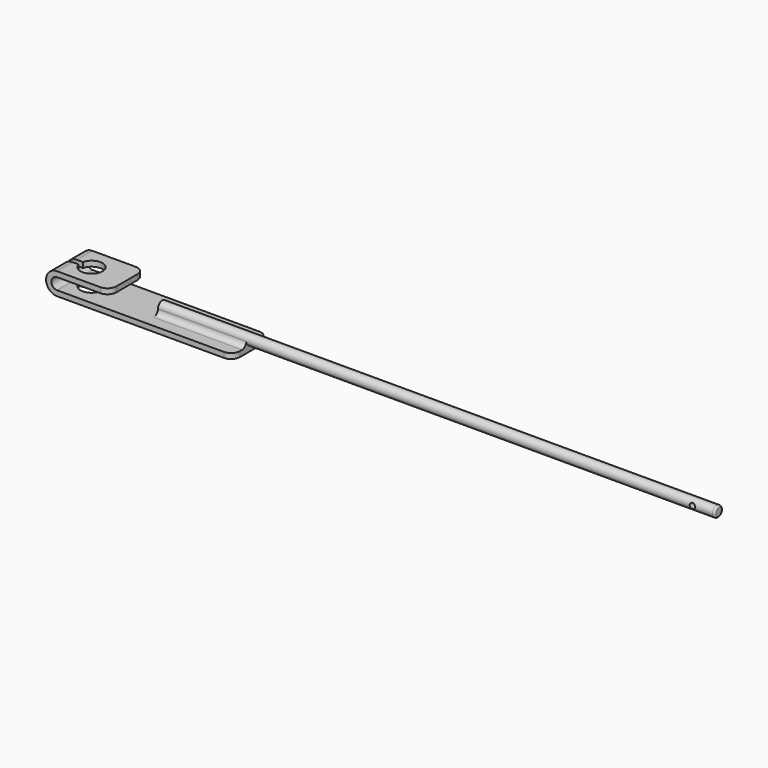
from build123d import *

# Parameters (mm, degrees)
F1_DEPTH      = 25
F3_DEPTH      = 12.501
F4_DEPTH      = 12.501
F7_DEPTH      = 270
F7_DEPTH_BACK = 45
F8_T1_DEPTH   = 45
F8_T3_DEPTH   = 5
F9_R          = 5
F10_R         = 1
F12_D         = 3


# Not quite as in the source:
# - a fillet or chamfer that OpenCascade refuses, or shapes differently, is made with other operations: its cross-section is extruded or revolved along the edge and cut away or added


with BuildPart() as f1:
    # F0 (on Front) → F1 (new body)
    with BuildSketch(Plane.XZ):
        with BuildLine():
            ThreePointArc((-35.5866095653, 3), (-41.8366095653, -3.25), (-35.5866095653, -9.5))
            Line((-35.5866095653, -9.5), (63.9133904347, -9.5))
            Line((63.9133904347, -9.5), (63.9133904347, -6.5))
            Line((63.9133904347, -6.5), (-35.5866095653, -6.5))
            ThreePointArc((-35.5866095653, -6.5), (-38.8366095653, -3.25), (-35.5866095653, 0))
            Line((-35.5866095653, 0), (-6.0866095653, 0))
            Line((-6.0866095653, 0), (-6.0866095653, 3))
            Line((-6.0866095653, 3), (-35.5866095653, 3))
        make_face()
    extrude(amount=F1_DEPTH)

    # F2 (on face) → F3 (cut, through all)
    with BuildSketch(Plane.XY.offset(3)):
        with BuildLine():
            ThreePointArc((-32.153940115, -14), (-25.3310686782, -18.7041645665), (-19.8366095653, -12.5))
            ThreePointArc((-19.8366095653, -12.5), (-25.3310686782, -6.2958354335), (-32.153940115, -11))
            ThreePointArc((-32.153940115, -11), (-32.3366095653, -12.5), (-32.153940115, -14))
        make_face()
    extrude(amount=-F3_DEPTH, mode=Mode.SUBTRACT)

    # F2 (on face) → F4 (cut, through all)
    with BuildSketch(Plane.XY.offset(3)):
        with BuildLine():
            ThreePointArc((-32.153940115, -14), (-25.3310686782, -18.7041645665), (-19.8366095653, -12.5))
            ThreePointArc((-19.8366095653, -12.5), (-25.3310686782, -6.2958354335), (-32.153940115, -11))
            ThreePointArc((-32.153940115, -11), (-32.3366095653, -12.5), (-32.153940115, -14))
        make_face()
        with BuildLine():
            ThreePointArc((-32.153940115, -14), (-32.3366095653, -12.5), (-32.153940115, -11))
            Line((-32.153940115, -11), (-41.9135839269, -11))
            Line((-41.9135839269, -11), (-41.9135839269, -14))
            Line((-41.9135839269, -14), (-32.153940115, -14))
        make_face()
    extrude(amount=-F4_DEPTH, mode=Mode.SUBTRACT)

    # F6 (on offset) → F7 (join, two sides)
    with BuildSketch(Plane.YZ.offset(58.9133904347)) as f7_sk:
        with BuildLine():
            ThreePointArc((-12.4225467883, -6.5), (-10.3514703126, -5.5947574316), (-9.5, -3.501))
            ThreePointArc((-9.5, -3.501), (-14.5937574316, -1.3524703126), (-12.5774532117, -6.5))
            Line((-12.5774532117, -6.5), (-12.4225467883, -6.5))
        make_face()
        with BuildLine():
            Line((-12.4225467883, -6.5), (-12.5774532117, -6.5))
            ThreePointArc((-12.5774532117, -6.5), (-12.5, -6.501), (-12.4225467883, -6.5))
        make_face()
    extrude(amount=F7_DEPTH)
    extrude(f7_sk.sketch, amount=-F7_DEPTH_BACK)

    # F8: fillet of radius 3 on 4 edges, made by hand

    # F8_s2 → F8_t1 (join)
    with BuildSketch(Plane.YZ.offset(13.9133904347)):
        with BuildLine():
            ThreePointArc((-18.5001459648, -6.5004), (-16.3786421293, -5.6217630236), (-15.4995999453, -3.5004270532))
            Line((-15.4995999453, -3.5004270532), (-15.1995453433, -3.500484366))
            ThreePointArc((-15.1995453433, -3.500484366), (-14.4336951193, -5.3852845615), (-12.5697064807, -6.2000454108))
            Line((-12.5697064807, -6.2000454108), (-12.5774532117, -6.8000546074))
            ThreePointArc((-12.5774532117, -6.8000546074), (-15.5387995882, -6.8000546074), (-18.5001459648, -6.8004546074))
            Line((-18.5001459648, -6.8004546074), (-18.5001459648, -6.5004))
        make_face()
        with BuildLine():
            ThreePointArc((-6.4998540352, -6.5004), (-8.6213578707, -5.6217630236), (-9.5004000547, -3.5004270532))
            Line((-9.5004000547, -3.5004270532), (-9.8004546567, -3.500484366))
            ThreePointArc((-9.8004546567, -3.500484366), (-10.5663048807, -5.3852845615), (-12.4302935193, -6.2000454108))
            Line((-12.4302935193, -6.2000454108), (-12.4225467883, -6.8000546074))
            ThreePointArc((-12.4225467883, -6.8000546074), (-9.4612004118, -6.8000546074), (-6.4998540352, -6.8004546074))
            Line((-6.4998540352, -6.8004546074), (-6.4998540352, -6.5004))
        make_face()
    extrude(amount=F8_T1_DEPTH)

    # F8_s4 → F8_t3 (join)
    with BuildSketch(Plane.YZ.offset(58.9133904347)):
        with BuildLine():
            ThreePointArc((-18.5001459648, -6.5004), (-16.3786421293, -5.6217630236), (-15.4995999453, -3.5004270532))
            Line((-15.4995999453, -3.5004270532), (-15.1995453433, -3.500484366))
            ThreePointArc((-15.1995453433, -3.500484366), (-14.4336951193, -5.3852845615), (-12.5697064807, -6.2000454108))
            Line((-12.5697064807, -6.2000454108), (-12.5774532117, -6.8000546074))
            ThreePointArc((-12.5774532117, -6.8000546074), (-15.5387995882, -6.8000546074), (-18.5001459648, -6.8004546074))
            Line((-18.5001459648, -6.8004546074), (-18.5001459648, -6.5004))
        make_face()
        with BuildLine():
            ThreePointArc((-6.4998540352, -6.5004), (-8.6213578707, -5.6217630236), (-9.5004000547, -3.5004270532))
            Line((-9.5004000547, -3.5004270532), (-9.8004546567, -3.500484366))
            ThreePointArc((-9.8004546567, -3.500484366), (-10.5663048807, -5.3852845615), (-12.4302935193, -6.2000454108))
            Line((-12.4302935193, -6.2000454108), (-12.4225467883, -6.8000546074))
            ThreePointArc((-12.4225467883, -6.8000546074), (-9.4612004118, -6.8000546074), (-6.4998540352, -6.8004546074))
            Line((-6.4998540352, -6.8004546074), (-6.4998540352, -6.5004))
        make_face()
    extrude(amount=F8_T3_DEPTH)

    # F9
    f9_edges = [f1.edges().sort_by_distance(p)[0] for p in [
        (63.91339, -25, -8),
        (63.91339, 0, -8),
        (-6.08661, 0, 1.5),
        (-6.08661, -25, 1.5),
    ]]
    fillet(f9_edges, radius=F9_R)

    # F10
    f10_edges = [f1.edges().sort_by_distance(p)[0] for p in [
        (328.91339, -15.5, -3.501),
    ]]
    fillet(f10_edges, radius=F10_R)

    # F12 (through all)
    with Locations(Plane(origin=(0, 0, 0), x_dir=(1, 0, 0), z_dir=(0, 1, 0))):
        with Locations((316.4133904347, 3.501)):
            Hole(F12_D / 2)


solid = f1.part
